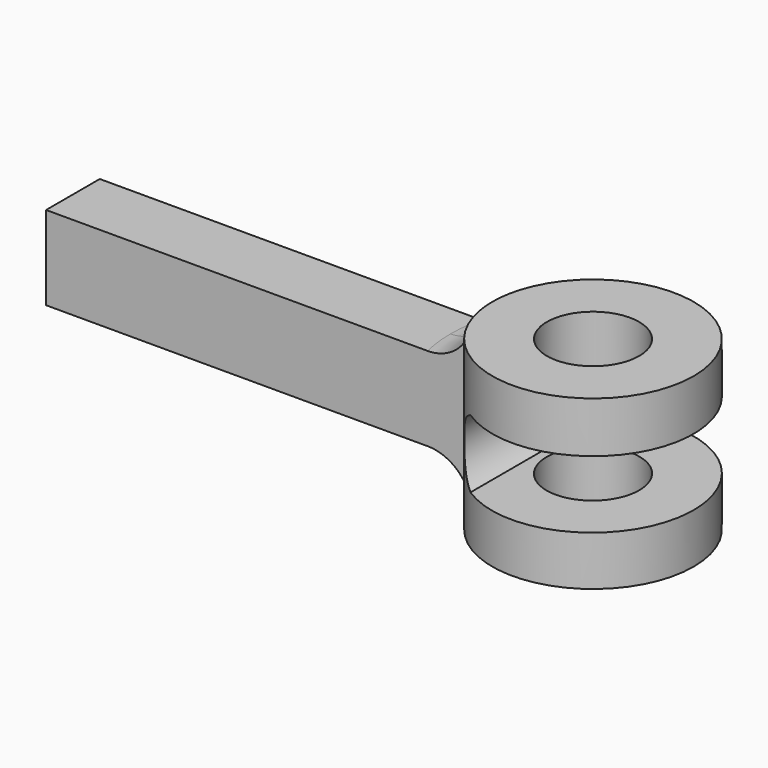
from build123d import *

# Parameters (mm, degrees)
F1_DEPTH      = 20
F1_DEPTH_BACK = 20
F3_DEPTH      = 10
F3_DEPTH_BACK = 10
F5_DEPTH      = 25
F5_DEPTH_BACK = 25
F6_T4_ANGLE   = 76.4346442218
F6_T10_ANGLE  = 76.4346442218
F6_T16_ANGLE  = 76.4346442218
F6_T22_ANGLE  = 76.4346442218


# Not quite as in the source:
# - a fillet or chamfer that OpenCascade refuses, or shapes differently, is made with other operations: its cross-section is extruded or revolved along the edge and cut away or added
# - two fillets or chamfers of one size are made in one step


with BuildPart() as f1:
    # F0 (on Top) → F1 (new body, two sides)
    with BuildSketch(Plane.XY) as f1_sk:
        with BuildLine():
            Line((11, 0), (24, 0))
            ThreePointArc((24, 0), (0, 24), (-24, 0))
            Line((-24, 0), (-11, 0))
            ThreePointArc((-11, 0), (0, 11), (11, 0))
        make_face()
        with BuildLine():
            ThreePointArc((-24, 0), (0, -24), (24, 0))
            Line((24, 0), (11, 0))
            ThreePointArc((11, 0), (0, -11), (-11, 0))
            Line((-11, 0), (-24, 0))
        make_face()
    extrude(amount=F1_DEPTH)
    extrude(f1_sk.sketch, amount=-F1_DEPTH_BACK)

    # F2 (on Top) → F3 (join, two sides)
    with BuildSketch(Plane.XY) as f3_sk:
        Polygon((-124.000001856, 8), (-124.000001856, 0), (-124.000001856, -8), (-22.981626913, -8), (-22.981626913, 8), align=None)
    extrude(amount=F3_DEPTH)
    extrude(f3_sk.sketch, amount=-F3_DEPTH_BACK)

    # F4 (on Front) → F5 (cut, two sides)
    with BuildSketch(Plane.XZ) as f5_sk:
        with BuildLine():
            Line((-13.159872964, -8.3219918372), (24.1259910374, -8.1159918464))
            Line((24.1259910374, -8.1159918464), (24.037594278, 7.8837639647))
            Line((24.037594278, 7.8837639647), (-13.159872964, 7.8837639647))
            ThreePointArc((-13.159872964, 7.8837639647), (-17.9421277203, -0.2191139363), (-13.159872964, -8.3219918372))
        make_face()
    extrude(amount=-F5_DEPTH, mode=Mode.SUBTRACT)
    extrude(f5_sk.sketch, amount=F5_DEPTH_BACK, mode=Mode.SUBTRACT)

    # F6: fillet of radius 10 on 4 edges, made by hand


with BuildPart() as f6_tool2:
    # F6_s3 → F6_t4 (revolve)
    with BuildSketch(Plane(origin=(0, 0, 0), x_dir=(0, 0, 1), z_dir=(0.9721030029, -0.2345543684, 0))):
        with BuildLine():
            ThreePointArc((20, 24), (12.9289321881, 26.9289321881), (10, 34))
            Line((10, 34), (10, 24))
            Line((10, 24), (20, 24))
        make_face()
    revolve(axis=Axis((0, 0, 10), (0, 0, -1)), revolution_arc=F6_T4_ANGLE)

    split(bisect_by=Plane.XZ.offset(8), keep=Keep.BOTTOM)

    split(bisect_by=Plane.YZ.offset(-22.981626913), keep=Keep.BOTTOM)


with BuildPart() as f1_1:
    add(f1.part)

    # F6_t1: union F6_tool2
    add(f6_tool2.part)


with BuildPart() as f6_tool8:
    # F6_s9 → F6_t10 (revolve)
    with BuildSketch(Plane.XZ):
        with BuildLine():
            ThreePointArc((-24, 20), (-26.9289321881, 12.9289321881), (-34, 10))
            Line((-34, 10), (-24, 10))
            Line((-24, 10), (-24, 20))
        make_face()
    revolve(axis=Axis((0, 0, 10), (0, 0, -1)), revolution_arc=F6_T10_ANGLE)

    split(bisect_by=Plane.XZ.offset(-8), keep=Keep.TOP)

    split(bisect_by=Plane.YZ.offset(-22.981626913), keep=Keep.BOTTOM)


with BuildPart() as f1_2:
    add(f1_1.part)

    # F6_t7: union F6_tool8
    add(f6_tool8.part)


with BuildPart() as f6_tool14:
    # F6_s15 → F6_t16 (revolve)
    with BuildSketch(Plane(origin=(0, 0, 0), x_dir=(0, 0, 1), z_dir=(0.9721030029, 0.2345543684, 0))):
        with BuildLine():
            ThreePointArc((-20, -24), (-12.9289321881, -26.9289321881), (-10, -34))
            Line((-10, -34), (-10, -24))
            Line((-10, -24), (-20, -24))
        make_face()
    revolve(axis=Axis((0, 0, -10), (0, 0, 1)), revolution_arc=F6_T16_ANGLE)

    split(bisect_by=Plane.XZ.offset(-8), keep=Keep.TOP)

    split(bisect_by=Plane.YZ.offset(-22.981626913), keep=Keep.BOTTOM)


with BuildPart() as f1_3:
    add(f1_2.part)

    # F6_t13: union F6_tool14
    add(f6_tool14.part)


with BuildPart() as f6_tool20:
    # F6_s21 → F6_t22 (revolve)
    with BuildSketch(Plane.XZ):
        with BuildLine():
            ThreePointArc((-24, -20), (-26.9289321881, -12.9289321881), (-34, -10))
            Line((-34, -10), (-24, -10))
            Line((-24, -10), (-24, -20))
        make_face()
    revolve(axis=Axis((0, 0, -10), (0, 0, 1)), revolution_arc=F6_T22_ANGLE)

    split(bisect_by=Plane.XZ.offset(8), keep=Keep.BOTTOM)

    split(bisect_by=Plane.YZ.offset(-22.981626913), keep=Keep.BOTTOM)


with BuildPart() as f1_4:
    add(f1_3.part)

    # F6_t19: union F6_tool20
    add(f6_tool20.part)


solid = f1_4.part
